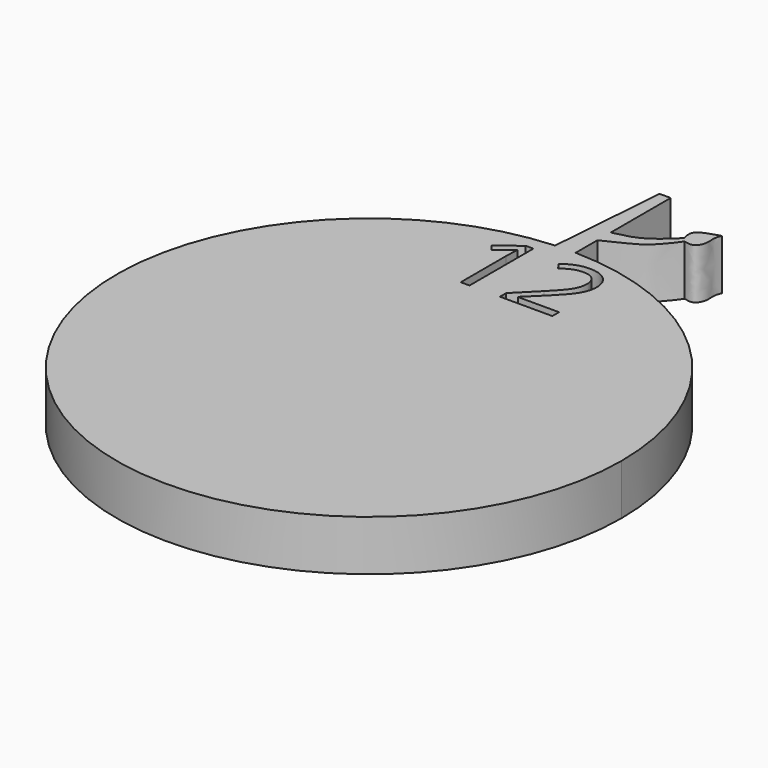
from build123d import *

# Parameters (mm, degrees)
F0_R         = 127
F1_DEPTH     = 25.4
F3_DEPTH     = 25.4
F5_DEPTH     = 25.4
F6_TEXT_SIZE = 56.2195873095
F7_DEPTH     = 50.8


# Not quite as in the source:
# - Text() gives the source's letters only with a copy of the font that has no kerning and outlines rounded to 1/6400 em; it was checked with that copy


with BuildPart() as f1:
    # F0 (on Top) → F1 (new body)
    with BuildSketch(Plane.XY):
        Circle(F0_R)
    extrude(amount=F1_DEPTH)

    # F2 (on Top) → F3 (join)
    with BuildSketch(Plane.XY):
        Polygon((-3.2720666661, 186.7402344942), (-7.8912936151, 125.9204298258), (2.3347195238, 125.1561790705), (2.3347195238, 186.7402344942), align=None)
    extrude(amount=F3_DEPTH)

    # F4 (on Top) → F5 (join)
    with BuildSketch(Plane.XY):
        with BuildLine():
            add(Edge.make_bspline(
                [(1.9974680617, 148.9690691233), (6.5400464023, 149.9389053809), (15.9863292236, 151.9556779919), (23.7478670979, 159.4684454983), (27.7769956738, 163.3684337139)],
                knots=[0, 0, 0, 0, 0.480885278, 1, 1, 1, 1], degree=3))
            add(Edge.make_bspline(
                [(1.9974680617, 148.9690691233), (1.8813441663, 146.0659652948), (1.7652202708, 143.1628614664), (1.6490963753, 140.259757638)],
                knots=[0, 0, 0, 0, 8.7162761188, 8.7162761188, 8.7162761188, 8.7162761188], degree=3))
            add(Edge.make_bspline(
                [(1.6490963753, 140.259757638), (7.7416428931, 143.3657663195), (15.6198525159, 146.7816729681), (22.659685025, 151.9509042506), (27.5964736717, 158.1932088478), (29.751105234, 161.2782031298)],
                knots=[0, 0, 0, 0, 0.3879654555, 0.6686610661, 1, 1, 1, 1], degree=3))
            add(Edge.make_bspline(
                [(29.751105234, 161.2782031298), (31.6778183639, 160.7570956344), (35.4452776234, 160.0253593365), (38.1532717763, 167.1641152587), (36.5116899969, 170.2447624947), (38.2229872048, 174.0951687098)],
                knots=[0, 0, 0, 0, 0.3045257595, 0.6238996936, 1, 1, 1, 1], degree=3))
            add(Edge.make_bspline(
                [(27.7769956738, 163.3684337139), (27.2658226838, 165.4925382979), (25.9632232396, 170.7330187755), (33.8238836183, 172.64559488), (38.2229872048, 174.0951687098)],
                knots=[0, 0, 0, 0, 0.4178228445, 1, 1, 1, 1], degree=3))
        make_face()
    extrude(amount=F5_DEPTH)

    # F6 (on face) → F7 (cut)
    with BuildSketch(Plane.XY.offset(25.4)):
        with Locations((-32.4580273607, 79.2246758938)):
            Text('12', F6_TEXT_SIZE, font='Open Sans', text_align=(TextAlign.LEFT, TextAlign.BOTTOM))
    extrude(amount=-F7_DEPTH, mode=Mode.SUBTRACT)


solid = f1.part
